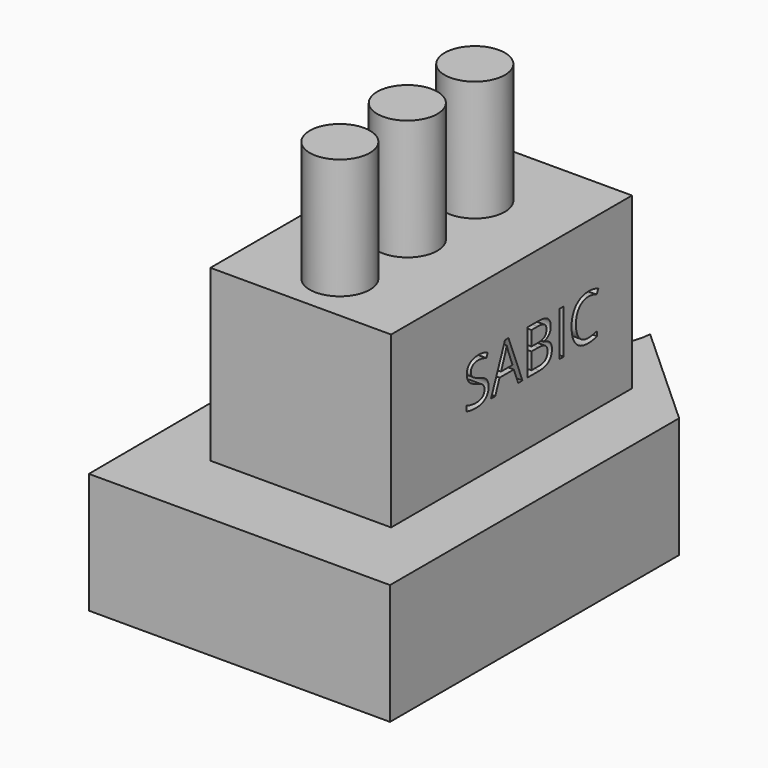
from build123d import *

# Parameters (mm, degrees)
F1_DEPTH     = 25.4
F2_W         = 38.1
F2_H         = 63.5
F3_DEPTH     = 35.814
F4_R         = 6.35
F5_DEPTH     = 25.4
F6_TEXT_SIZE = 13.0934744245
F7_DEPTH     = 47.498
F8_R         = 11.9977628717
F9_DEPTH     = 25.4


# Not quite as in the source:
# - Text() gives the source's letters only with a copy of the font that has no kerning and outlines rounded to 1/6400 em; it was checked with that copy


with BuildPart() as f1:
    # F0 (on Top) → F1 (new body)
    with BuildSketch(Plane.XY):
        Polygon((-32.0597537315, 31.9548403475), (-31.75, -44.244530074), (31.75, -44.244530074), (31.75, 31.955469926), (0, 60.8370981488), align=None)
    extrude(amount=F1_DEPTH)

    # F2 (on face) → F3 (join)
    with BuildSketch(Plane.XY.offset(25.4)):
        with Locations((0, 3.6617376797)):
            Rectangle(F2_W, F2_H)
    extrude(amount=F3_DEPTH)

    # F4 (on face) → F5 (join)
    with BuildSketch(Plane.XY.offset(61.214)):
        with Locations((0, 17.78)):
            Circle(F4_R)
        Circle(F4_R)
        with Locations((0, -17.78)):
            Circle(F4_R)
    extrude(amount=F5_DEPTH)

    # F6 (on face) → F7 (cut)
    with BuildSketch(Plane.YZ.offset(19.05)):
        with Locations((-8.9355027303, 38.6026725173)):
            Text('SABIC', F6_TEXT_SIZE, font='Open Sans', text_align=(TextAlign.LEFT, TextAlign.BOTTOM))
    extrude(amount=-F7_DEPTH, mode=Mode.SUBTRACT)

    # F8 (on face) → F9 (cut)
    with BuildSketch(Plane.XY.offset(25.4)):
        with Locations((-2.6827815454, 53.0243776739)):
            Circle(F8_R)
    extrude(amount=-F9_DEPTH, mode=Mode.SUBTRACT)


solid = f1.part
